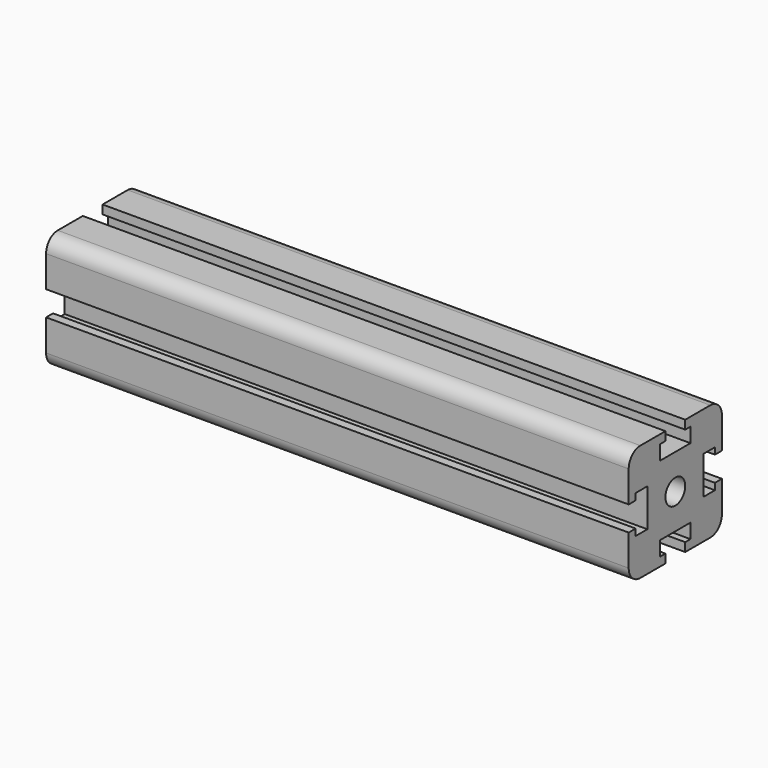
from build123d import *

# Parameters (mm, degrees)
F0_W            = 40
F0_H            = 40
F1_DEPTH        = 200
F3_DEPTH        = 200
F3_COPIES_COUNT = 4
F4_R            = 5
F5_R            = 4.25
F6_DEPTH        = 200


# Not quite as in the source:
# - a pattern or mirror of a feature is missing from the dataset's text; its kind, count and spacing are read off the source's solid


with BuildPart() as f1:
    # F0 (on Right) → F1 (new body)
    with BuildSketch(Plane.YZ):
        Rectangle(F0_W, F0_H)
    extrude(amount=F1_DEPTH)

    # F2 (on face) → F3 (cut, through all)
    with BuildSketch(Plane.YZ.offset(200)):
        Polygon((4.25, 20), (-4.25, 20), (-4.25, 17), (-6.5, 17), (-6.5, 12), (6.5, 12), (6.5, 17), (4.25, 17), align=None)
    f3 = extrude(amount=-F3_DEPTH, mode=Mode.SUBTRACT)

    # F3_copies: F3 ×4 about axis
    f3_copies_axis = Axis((0, 0, 0), (1, 0, 0))
    for i in range(1, F3_COPIES_COUNT):
        add(f3.rotate(f3_copies_axis, i * 360 / F3_COPIES_COUNT), mode=Mode.SUBTRACT)

    # F4
    f4_edges = [f1.edges().sort_by_distance(p)[0] for p in [
        (100, 20, 20),
        (100, -20, 20),
        (100, 20, -20),
        (100, -20, -20),
    ]]
    fillet(f4_edges, radius=F4_R)

    # F5 (on face) → F6 (cut, through all)
    with BuildSketch(Plane.YZ.offset(200)):
        Circle(F5_R)
    extrude(amount=-F6_DEPTH, mode=Mode.SUBTRACT)


solid = f1.part
